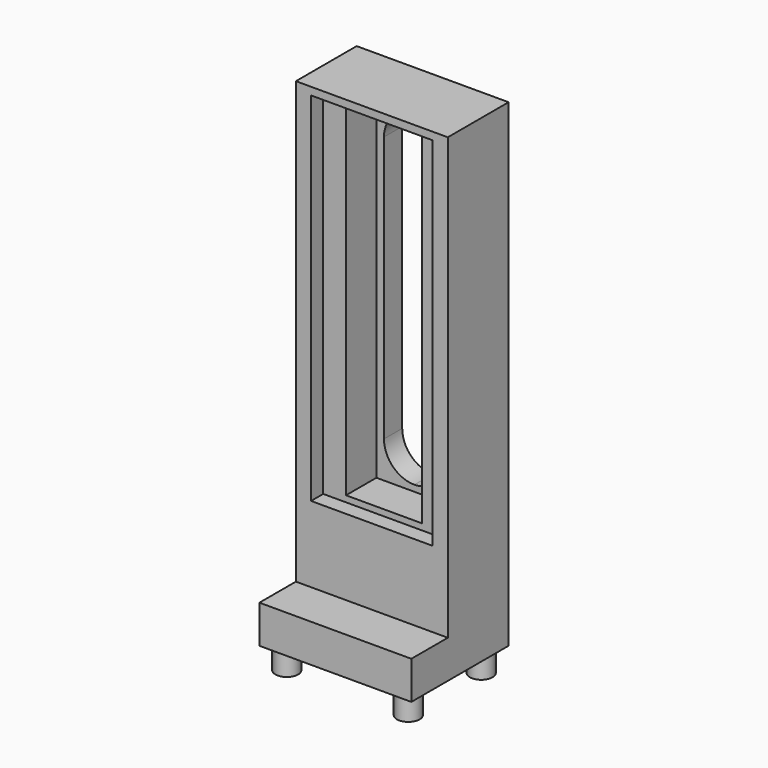
from build123d import *

# Parameters (mm, degrees)
F0_W     = 254
F0_H     = 736.6
F0_W_2   = 203.2
F0_H_2   = 596.9
F0_W_3   = 127
F0_H_3   = 571.5
F0_W_4   = 101.6
F0_H_4   = 546.1
F0_H_5   = 63.5
F1_DEPTH = 127
F2_DEPTH = 25.4
F3_DEPTH = 88.9
F4_R     = 50.79999
F5_DEPTH = 76.2
F6_R     = 19.05
F7_DEPTH = 38.1


# Not quite as in the source:
# - a fillet or chamfer is up to 0.001 mm smaller than in the source, because OpenCascade refuses the exact size
# - a feature names something its author has since deleted; it is built from what else it names


with BuildPart() as f1:
    # F0 (on Front) → F1 (new body)
    with BuildSketch(Plane.XZ):
        with Locations((0, 241.3)):
            Rectangle(F0_W, F0_H)
        with Locations((0, 298.45)):
            Rectangle(F0_W_2, F0_H_2, mode=Mode.SUBTRACT)
        with Locations((0, 298.45)):
            Rectangle(F0_W_2, F0_H_2)
        with Locations((0, 296.15)):
            Rectangle(F0_W_3, F0_H_3, mode=Mode.SUBTRACT)
        with Locations((0, 296.15)):
            Rectangle(F0_W_3, F0_H_3)
        with Locations((0, 293.85)):
            Rectangle(F0_W_4, F0_H_4, mode=Mode.SUBTRACT)
        with Locations((0, -158.75)):
            Rectangle(F0_W, F0_H_5)
    extrude(amount=-F1_DEPTH)

    # F0 (on Front) → F2 (cut)
    with BuildSketch(Plane.XZ):
        with Locations((0, 298.45)):
            Rectangle(F0_W_2, F0_H_2)
        with Locations((0, 296.15)):
            Rectangle(F0_W_3, F0_H_3, mode=Mode.SUBTRACT)
    extrude(amount=-F2_DEPTH, mode=Mode.SUBTRACT)

    # F0 (on Front) → F3 (cut)
    with BuildSketch(Plane.XZ):
        with Locations((0, 296.15)):
            Rectangle(F0_W_3, F0_H_3)
        with Locations((0, 293.85)):
            Rectangle(F0_W_4, F0_H_4, mode=Mode.SUBTRACT)
    extrude(amount=-F3_DEPTH, mode=Mode.SUBTRACT)

    # F4 (radius 50.8 in the source; OpenCascade refuses exactly that, so slightly less here)
    f4_edges = [f1.edges().sort_by_distance(p)[0] for p in [
        (50.8, 107.95, 566.9),
        (-50.8, 107.95, 566.9),
        (-50.8, 107.95, 20.8),
        (50.8, 107.95, 20.8),
    ]]
    fillet(f4_edges, radius=F4_R)

    # F0 (on Front) → F5 (join)
    with BuildSketch(Plane.XZ):
        with Locations((0, -158.75)):
            Rectangle(F0_W, F0_H_5)
    extrude(amount=F5_DEPTH)

    # F6 (on face) → F7 (join)
    with BuildSketch(Plane(origin=(0, 0, -190.5), x_dir=(1, 0, 0), z_dir=(0, 0, -1))):
        with Locations((-101.6, 50.8)):
            Circle(F6_R)
        with Locations((101.6, 50.8)):
            Circle(F6_R)
        with Locations((-101.6, -101.6)):
            Circle(F6_R)
        with Locations((101.6, -101.6)):
            Circle(F6_R)
    extrude(amount=F7_DEPTH)


solid = f1.part
